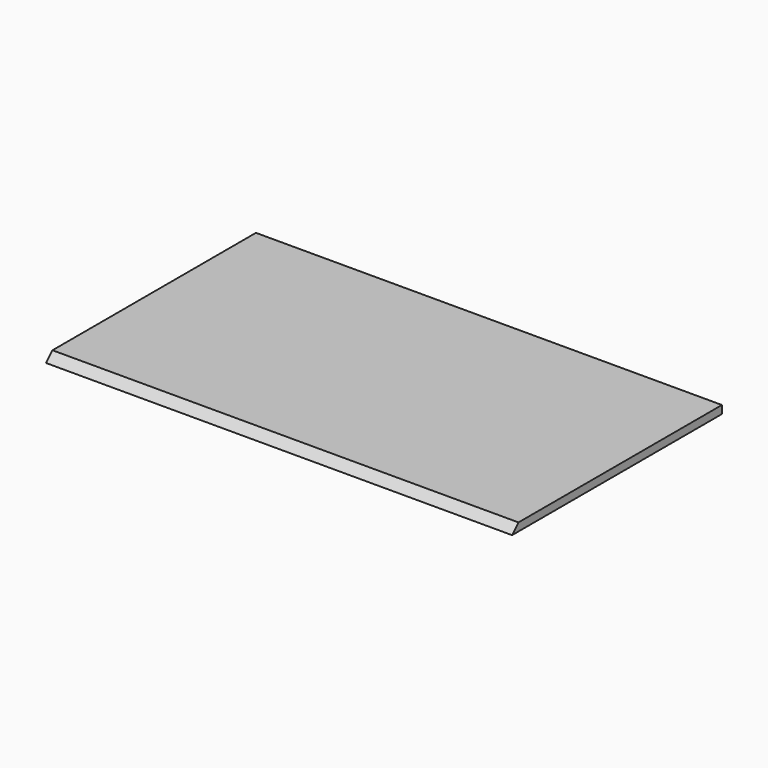
from build123d import *

# Parameters (mm, degrees)
F0_W     = 350
F0_H     = 200
F1_DEPTH = 6
F2_SIZE  = 5.99999
F3_DEPTH = 3


# Not quite as in the source:
# - a fillet or chamfer is up to 0.001 mm smaller than in the source, because OpenCascade refuses the exact size


with BuildPart() as f1:
    # F0 (on Top) → F1 (new body)
    with BuildSketch(Plane.XY):
        with Locations((103.189206589, -5.372708199)):
            Rectangle(F0_W, F0_H)
    extrude(amount=F1_DEPTH)

    # F2 (size 6 in the source; OpenCascade refuses exactly that, so slightly less here)
    f2_edges = [f1.edges().sort_by_distance(p)[0] for p in [
        (103.189207, -105.372708, 6),
    ]]
    chamfer(f2_edges, length=F2_SIZE)

    # F3 (cut): a face of the model
    f3_faces = [f1.faces().sort_by_distance(p)[0] for p in [
        (103.189206589, 94.627291801, 3),
    ]]
    extrude(f3_faces, amount=-F3_DEPTH, mode=Mode.SUBTRACT)


solid = f1.part
